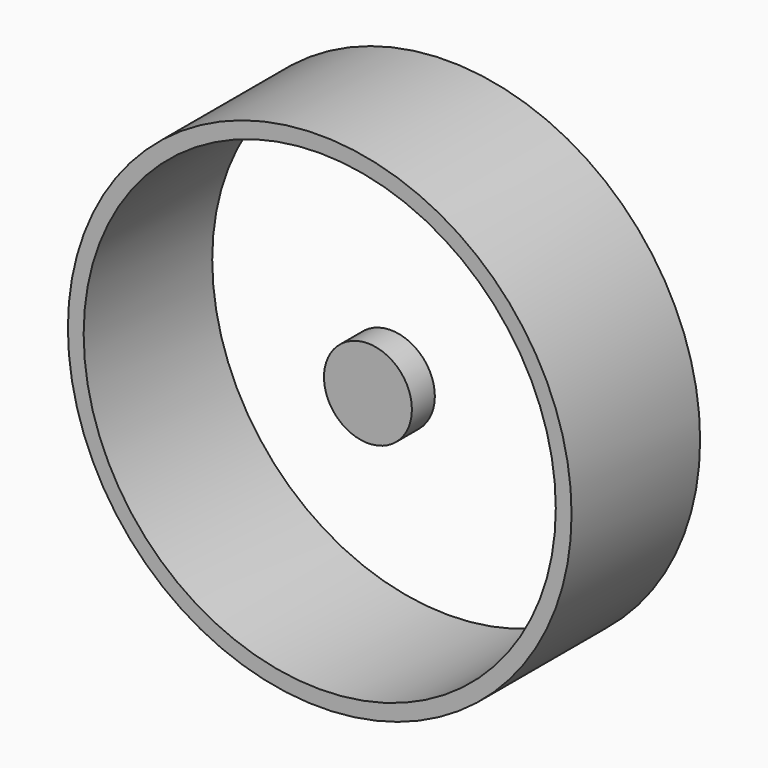
from build123d import *

# Parameters (mm, degrees)
F0_R     = 7.6609031883
F1_DEPTH = 5
F2_R     = 43.8831518485
F2_R_2   = 41.1346697105
F3_DEPTH = 15.5
F4_DEPTH = 25
F5_DEPTH = 12.5


# Not quite as in the source:
# - the program builds the solid bodies; features that only make, move or delete a surface that nothing else refers to are left out


with BuildPart() as f1:
    # F0 (on Front) → F1 (new body)
    with BuildSketch(Plane.XZ):
        Circle(F0_R)
    extrude(amount=F1_DEPTH)


with BuildPart() as f3:
    # F2 (on Front) → F3 (new body, symmetric)
    with BuildSketch(Plane.XZ):
        Circle(F2_R)
        Circle(F2_R_2, mode=Mode.SUBTRACT)
    extrude(amount=F3_DEPTH, both=True)

    # F2 (on Front) → F4 (cut)
    with BuildSketch(Plane.XZ):
        Circle(F2_R)
        Circle(F2_R_2, mode=Mode.SUBTRACT)
    extrude(amount=-F4_DEPTH, mode=Mode.SUBTRACT)

    # F2 (on Front) → F5 (join, symmetric)
    with BuildSketch(Plane.XZ):
        Circle(F2_R)
        Circle(F2_R_2, mode=Mode.SUBTRACT)
    extrude(amount=F5_DEPTH, both=True)


solid = Compound([f1.part, f3.part])
